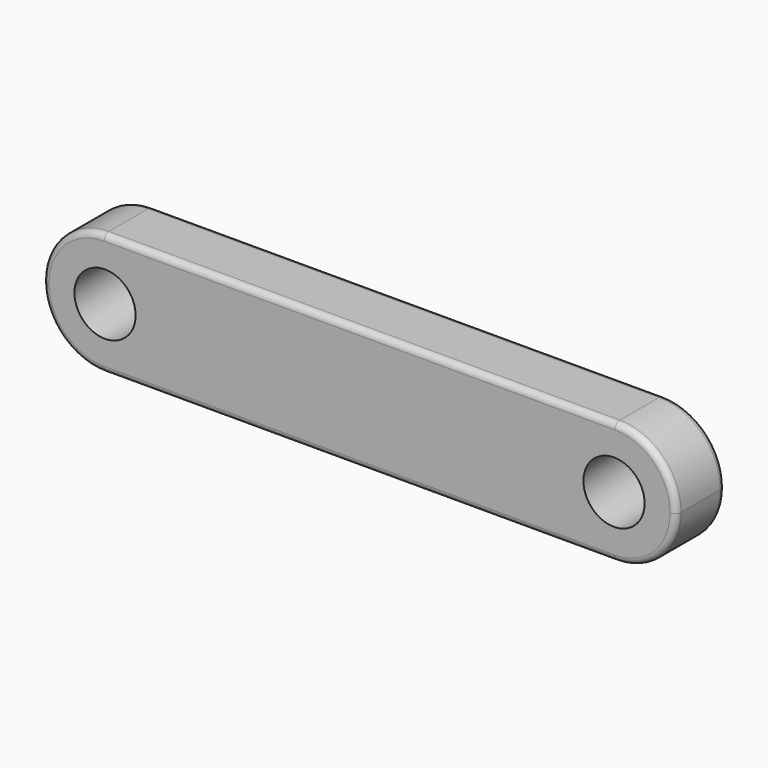
from build123d import *

# Parameters (mm, degrees)
F0_W     = 20.7
F0_H     = 4
F1_DEPTH = 2
F2_R     = 1.99999
F3_R     = 0.2
F4_R     = 1
F5_DEPTH = 25


# Not quite as in the source:
# - a fillet or chamfer is up to 0.001 mm smaller than in the source, because OpenCascade refuses the exact size


with BuildPart() as f1:
    # F0 (on Front) → F1 (new body)
    with BuildSketch(Plane.XZ):
        with Locations((-0.2598203719, 2.9809341038)):
            Rectangle(F0_W, F0_H)
    extrude(amount=F1_DEPTH)

    # F2 (radius 2 in the source; OpenCascade refuses exactly that, so slightly less here)
    f2_edges = [f1.edges().sort_by_distance(p)[0] for p in [
        (-10.60982, -1, 4.980934),
        (-10.60982, -1, 0.980934),
        (10.09018, -1, 4.980934),
        (10.09018, -1, 0.980934),
    ]]
    fillet(f2_edges, radius=F2_R)

    # F3
    f3_edges = [f1.edges().sort_by_distance(p)[0] for p in [
        (-0.25982, 0, 4.980934),
        (-0.25982, -2, 4.980934),
    ]]
    fillet(f3_edges, radius=F3_R)

    # F4 (on face) → F5 (cut)
    with BuildSketch(Plane(origin=(0, 0, 0), x_dir=(-1, 0, 0), z_dir=(0, 1, 0))):
        with Locations((8.5788203719, 2.9809341038)):
            Circle(F4_R)
        with Locations((-8.0591796281, 2.9809341038)):
            Circle(F4_R)
    extrude(amount=-F5_DEPTH, mode=Mode.SUBTRACT)


solid = f1.part
